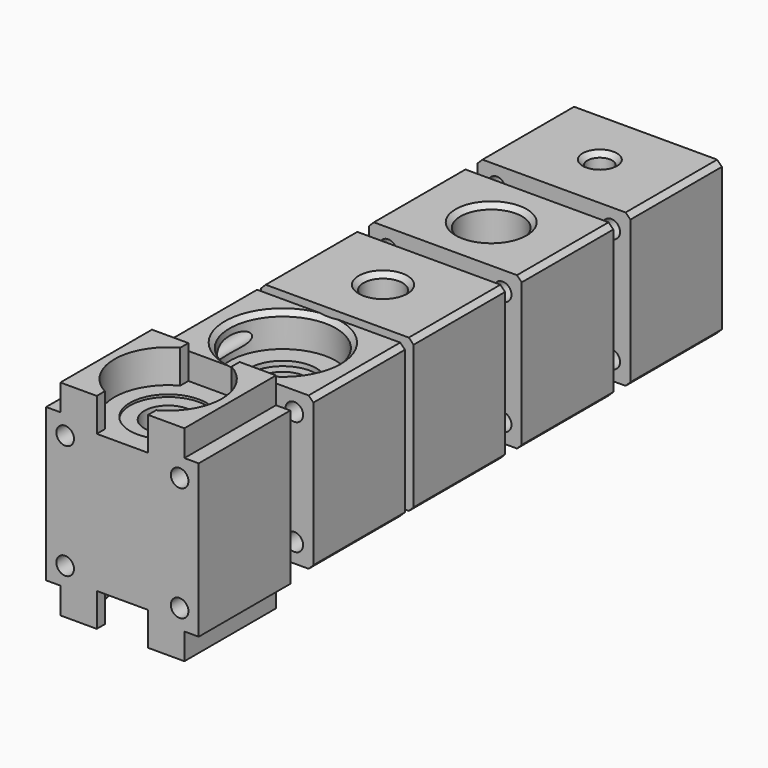
from build123d import *

# Parameters (mm, degrees)
F0_W          = 32
F0_H          = 24
F0_R          = 11.15
F0_R_2        = 7
F0_R_3        = 5
F1_DEPTH      = 32
F0_R_4        = 4.1
F0_R_5        = 6.45
F0_R_6        = 2.6
F2_R          = 1.85
F3_DEPTH      = 125.12902881
F4_R          = 11.15
F4_R_2        = 7
F5_DEPTH      = 7
F6_DEPTH      = 7
F7_C1_SIZE    = 1
F7_C2_SIZE    = 1
F7_C3_SIZE    = 1
F7_C4_SIZE    = 1
F7_C5_SIZE    = 1
F7_C6_SIZE    = 1
F7_2_C1_SIZE  = 1
F7_2_C2_SIZE  = 1
F7_2_C3_SIZE  = 1
F7_2_C4_SIZE  = 1
F7_2_C5_SIZE  = 1
F7_2_C6_SIZE  = 1
F7_3_C1_SIZE  = 1
F7_3_C2_SIZE  = 1
F7_3_C3_SIZE  = 1
F7_3_C4_SIZE  = 1
F7_3_C5_SIZE  = 1
F7_3_C6_SIZE  = 1
F7_4_T1_DEPTH = 29.1433659759
F8_DEPTH      = 8
F9_DEPTH      = 8
F10_R         = 1.85
F11_DEPTH     = 12
F14_DEPTH     = 7
F15_W         = 10.7521517202
F15_H         = 26.6113560647
F16_DEPTH     = 7


# Not quite as in the source:
# - a fillet or chamfer that OpenCascade refuses, or shapes differently, is made with other operations: its cross-section is extruded or revolved along the edge and cut away or added


with BuildPart() as f1:
    # F0 (on Top) → F1 (new body)
    with BuildSketch(Plane.XY):
        with Locations((0, 30.0521291792)):
            Rectangle(F0_W, F0_H)
        with Locations((0, 30.0521291792)):
            Circle(F0_R, mode=Mode.SUBTRACT)
        with Locations((0, 30.0521291792)):
            Circle(F0_R)
        with Locations((0, 30.0521291792)):
            Circle(F0_R_2, mode=Mode.SUBTRACT)
        with Locations((0, 30.0521291792)):
            Circle(F0_R_2)
        with Locations((0, 30.0521291792)):
            Circle(F0_R_3, mode=Mode.SUBTRACT)
    extrude(amount=F1_DEPTH)


with BuildPart() as f1b:
    # F0 (on Top) → F1, piece 2 (new body)
    with BuildSketch(Plane.XY):
        with Locations((0, 56.3173405826)):
            Rectangle(F0_W, F0_H)
        with Locations((0, 56.3173405826)):
            Circle(F0_R_4, mode=Mode.SUBTRACT)
    extrude(amount=F1_DEPTH)


with BuildPart() as f1c:
    # F0 (on Top) → F1, piece 3 (new body)
    with BuildSketch(Plane.XY):
        with Locations((0, 84.6606269479)):
            Rectangle(F0_W, F0_H)
        with Locations((0, 84.6606269479)):
            Circle(F0_R_5, mode=Mode.SUBTRACT)
    extrude(amount=F1_DEPTH)


with BuildPart() as f1d:
    # F0 (on Top) → F1, piece 4 (new body)
    with BuildSketch(Plane.XY):
        with Locations((0, 113.12802881)):
            Rectangle(F0_W, F0_H)
        with Locations((0, 113.12802881)):
            Circle(F0_R_6, mode=Mode.SUBTRACT)
    extrude(amount=F1_DEPTH)


with BuildPart() as f3_tool:
    # F2 (on Front) → F3 (new body, through all)
    with BuildSketch(Plane.XZ):
        with Locations((-12, 28)):
            Circle(F2_R)
        with Locations((12, 28)):
            Circle(F2_R)
        with Locations((12, 4)):
            Circle(F2_R)
        with Locations((-12, 4)):
            Circle(F2_R)
    extrude(amount=-F3_DEPTH)


with BuildPart() as f1_1:
    add(f1.part)

    # F3: cut by f3_tool
    add(f3_tool.part, mode=Mode.SUBTRACT)

    # F4 (on face) → F5 (cut)
    with BuildSketch(Plane.XY.offset(32)):
        with Locations((0, 30.0521291792)):
            Circle(F4_R)
        with Locations((0, 30.0521291792)):
            Circle(F4_R_2, mode=Mode.SUBTRACT)
    extrude(amount=-F5_DEPTH, mode=Mode.SUBTRACT)

    # F0 (on Top) → F6 (cut)
    with BuildSketch(Plane.XY):
        with Locations((0, 30.0521291792)):
            Circle(F0_R)
        with Locations((0, 30.0521291792)):
            Circle(F0_R_2, mode=Mode.SUBTRACT)
    extrude(amount=F6_DEPTH, mode=Mode.SUBTRACT)

    # F7#4: chamfer of 1 on 6 edges, made by hand

    # F7_4_s2 → F7_4_t1 (cut)
    with BuildSketch(Plane.XZ.offset(-44.6238121672)):
        Polygon((15, 32), (16, 31), (16, 32), align=None)
        Polygon((-16, 31), (-15, 32), (-16, 32), align=None)
        Polygon((15, 0), (16, 1), (16, 0), align=None)
        Polygon((-16, 1), (-15, 0), (-16, 0), align=None)
    extrude(amount=F7_4_T1_DEPTH, mode=Mode.SUBTRACT)

    # F7_4_s3 → F7_4_t4 (revolve, cut)
    with BuildSketch(Plane.XZ.offset(-30.0521291792)):
        Polygon((12.15, 32), (11.15, 31), (11.15, 32), align=None)
    revolve(axis=Axis((0, 30.0521291792, 32), (0, 0, 1)), mode=Mode.SUBTRACT)

    # F7_4_s5 → F7_4_t6 (revolve, cut)
    with BuildSketch(Plane.XZ.offset(-30.0521291792)):
        Polygon((12.15, 0), (11.15, 1), (11.15, 0), align=None)
    revolve(axis=Axis((0, 30.0521291792, 0), (0, 0, 1)), mode=Mode.SUBTRACT)

    # F0 (on Top) → F8 (cut)
    with BuildSketch(Plane.XY):
        with Locations((0, 30.0521291792)):
            Circle(F0_R_2)
        with Locations((0, 30.0521291792)):
            Circle(F0_R_3, mode=Mode.SUBTRACT)
    extrude(amount=F8_DEPTH, mode=Mode.SUBTRACT)

    # F9 (cut): a face of the model
    f9_faces = [f1_1.faces().sort_by_distance(p)[0] for p in [
        (-6.8020101013, 30.0521291792, 32),
    ]]
    extrude(f9_faces, amount=-F9_DEPTH, mode=Mode.SUBTRACT)


with BuildPart() as f1b_1:
    add(f1b.part)

    # F3: cut by f3_tool
    add(f3_tool.part, mode=Mode.SUBTRACT)

    # F7#3: chamfer of 1 on 6 edges, made by hand

    # F7_3_c1
    f7_3_c1_edges = [f1b_1.edges().sort_by_distance(p)[0] for p in [
        (-16, 56.3173405826, 0),
    ]]
    chamfer(f7_3_c1_edges, length=F7_3_C1_SIZE)

    # F7_3_c2
    f7_3_c2_edges = [f1b_1.edges().sort_by_distance(p)[0] for p in [
        (-16, 56.3173405826, 32),
    ]]
    chamfer(f7_3_c2_edges, length=F7_3_C2_SIZE)

    # F7_3_c3
    f7_3_c3_edges = [f1b_1.edges().sort_by_distance(p)[0] for p in [
        (16, 56.3173405826, 0),
    ]]
    chamfer(f7_3_c3_edges, length=F7_3_C3_SIZE)

    # F7_3_c4
    f7_3_c4_edges = [f1b_1.edges().sort_by_distance(p)[0] for p in [
        (-4.1, 56.3173405826, 0),
    ]]
    chamfer(f7_3_c4_edges, length=F7_3_C4_SIZE)

    # F7_3_c5
    f7_3_c5_edges = [f1b_1.edges().sort_by_distance(p)[0] for p in [
        (16, 56.3173405826, 32),
    ]]
    chamfer(f7_3_c5_edges, length=F7_3_C5_SIZE)

    # F7_3_c6
    f7_3_c6_edges = [f1b_1.edges().sort_by_distance(p)[0] for p in [
        (-4.1, 56.3173405826, 32),
    ]]
    chamfer(f7_3_c6_edges, length=F7_3_C6_SIZE)


with BuildPart() as f1c_1:
    add(f1c.part)

    # F3: cut by f3_tool
    add(f3_tool.part, mode=Mode.SUBTRACT)

    # F7#2: chamfer of 1 on 6 edges, made by hand

    # F7_2_c1
    f7_2_c1_edges = [f1c_1.edges().sort_by_distance(p)[0] for p in [
        (-16, 84.6606269479, 0),
    ]]
    chamfer(f7_2_c1_edges, length=F7_2_C1_SIZE)

    # F7_2_c2
    f7_2_c2_edges = [f1c_1.edges().sort_by_distance(p)[0] for p in [
        (-16, 84.6606269479, 32),
    ]]
    chamfer(f7_2_c2_edges, length=F7_2_C2_SIZE)

    # F7_2_c3
    f7_2_c3_edges = [f1c_1.edges().sort_by_distance(p)[0] for p in [
        (16, 84.6606269479, 0),
    ]]
    chamfer(f7_2_c3_edges, length=F7_2_C3_SIZE)

    # F7_2_c4
    f7_2_c4_edges = [f1c_1.edges().sort_by_distance(p)[0] for p in [
        (-6.45, 84.6606269479, 0),
    ]]
    chamfer(f7_2_c4_edges, length=F7_2_C4_SIZE)

    # F7_2_c5
    f7_2_c5_edges = [f1c_1.edges().sort_by_distance(p)[0] for p in [
        (16, 84.6606269479, 32),
    ]]
    chamfer(f7_2_c5_edges, length=F7_2_C5_SIZE)

    # F7_2_c6
    f7_2_c6_edges = [f1c_1.edges().sort_by_distance(p)[0] for p in [
        (-6.45, 84.6606269479, 32),
    ]]
    chamfer(f7_2_c6_edges, length=F7_2_C6_SIZE)


with BuildPart() as f1d_1:
    add(f1d.part)

    # F3: cut by f3_tool
    add(f3_tool.part, mode=Mode.SUBTRACT)

    # F7: chamfer of 1 on 6 edges, made by hand

    # F7_c1
    f7_c1_edges = [f1d_1.edges().sort_by_distance(p)[0] for p in [
        (-16, 113.12802881, 0),
    ]]
    chamfer(f7_c1_edges, length=F7_C1_SIZE)

    # F7_c2
    f7_c2_edges = [f1d_1.edges().sort_by_distance(p)[0] for p in [
        (-16, 113.12802881, 32),
    ]]
    chamfer(f7_c2_edges, length=F7_C2_SIZE)

    # F7_c3
    f7_c3_edges = [f1d_1.edges().sort_by_distance(p)[0] for p in [
        (16, 113.12802881, 0),
    ]]
    chamfer(f7_c3_edges, length=F7_C3_SIZE)

    # F7_c4
    f7_c4_edges = [f1d_1.edges().sort_by_distance(p)[0] for p in [
        (-2.6, 113.12802881, 0),
    ]]
    chamfer(f7_c4_edges, length=F7_C4_SIZE)

    # F7_c5
    f7_c5_edges = [f1d_1.edges().sort_by_distance(p)[0] for p in [
        (16, 113.12802881, 32),
    ]]
    chamfer(f7_c5_edges, length=F7_C5_SIZE)

    # F7_c6
    f7_c6_edges = [f1d_1.edges().sort_by_distance(p)[0] for p in [
        (-2.6, 113.12802881, 32),
    ]]
    chamfer(f7_c6_edges, length=F7_C6_SIZE)


with BuildPart() as f11:
    # F10 (on Front) → F11 (new body, symmetric)
    with BuildSketch(Plane.XZ):
        Polygon((-16, 32), (-16, 0), (-13, 0), (-13, -5.5), (0, -5.5), (0, 37.5), (-13, 37.5), (-13, 32), align=None)
        with Locations((-12, 4)):
            Circle(F10_R, mode=Mode.SUBTRACT)
        with Locations((-12, 28)):
            Circle(F10_R, mode=Mode.SUBTRACT)
        Polygon((0, 37.5), (0, -5.5), (11.25, -5.5), (11.25, 1.5), (8, 1.5), (8, 2), (5, 2), (5, 30), (8, 30), (8, 30.5), (11.25, 30.5), (11.25, 37.5), align=None)
        Polygon((11.25, 1.5), (11.25, -5.5), (13, -5.5), (13, 0), (16, 0), (16, 32), (13, 32), (13, 37.5), (11.25, 37.5), (11.25, 30.5), (8, 30.5), (8, 30), (5, 30), (5, 2), (8, 2), (8, 1.5), align=None)
        with Locations((12, 4)):
            Circle(F10_R, mode=Mode.SUBTRACT)
        with Locations((12, 28)):
            Circle(F10_R, mode=Mode.SUBTRACT)
    extrude(amount=F11_DEPTH, both=True)

    # F10 (on Front) → F12 (revolve, cut)
    with BuildSketch(Plane.XZ):
        Polygon((0, 37.5), (0, -5.5), (11.25, -5.5), (11.25, 1.5), (8, 1.5), (8, 2), (5, 2), (5, 30), (8, 30), (8, 30.5), (11.25, 30.5), (11.25, 37.5), align=None)
    revolve(axis=Axis((0, 0, 16), (0, 0, -1)), mode=Mode.SUBTRACT)

    # F13 (on face) → F14 (cut)
    with BuildSketch(Plane.XY.offset(37.5)):
        with BuildLine():
            ThreePointArc((-5.3760758601, 9.8823230238), (0, 11.25), (5.3760758601, 9.8823230238))
            Line((5.3760758601, 9.8823230238), (5.3760758601, 12))
            Line((5.3760758601, 12), (-5.3760758601, 12))
            Line((-5.3760758601, 12), (-5.3760758601, 9.8823230238))
        make_face()
        with BuildLine():
            Line((-5.3760758601, -12), (5.3760758601, -12))
            Line((5.3760758601, -12), (5.3760758601, -9.8823230238))
            ThreePointArc((5.3760758601, -9.8823230238), (0, -11.25), (-5.3760758601, -9.8823230238))
            Line((-5.3760758601, -9.8823230238), (-5.3760758601, -12))
        make_face()
    extrude(amount=-F14_DEPTH, mode=Mode.SUBTRACT)

    # F15 (on face) → F16 (cut)
    with BuildSketch(Plane(origin=(0, 0, -5.5), x_dir=(1, 0, 0), z_dir=(0, 0, -1))):
        Rectangle(F15_W, F15_H)
    extrude(amount=-F16_DEPTH, mode=Mode.SUBTRACT)


solid = Compound([f1_1.part, f1b_1.part, f1c_1.part, f1d_1.part, f11.part])
